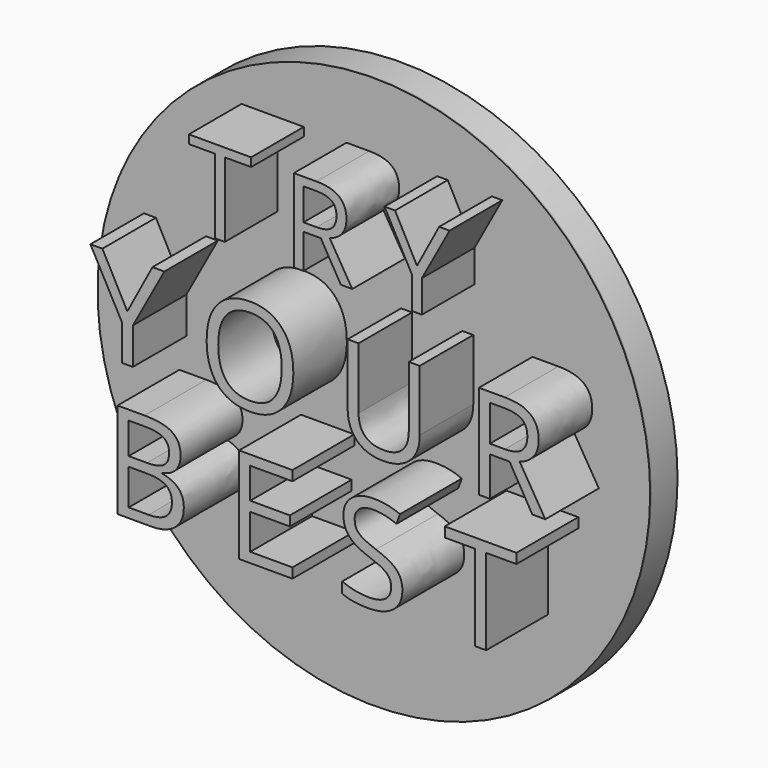
from build123d import *

# Parameters (mm, degrees)
F0_R         = 74.7496845117
F1_DEPTH     = 9.25076
F2_DEPTH     = 8.89276
F3_TEXT_SIZE = 31.4468880081
F6_DEPTH     = 17.81762
F4_TEXT_SIZE = 35.690900404
F7_DEPTH     = 18.10013
F5_TEXT_SIZE = 36.2257731871
F8_DEPTH     = 20.90356


# Not quite as in the source:
# - Text() gives the source's letters only with a copy of the font that has no kerning and outlines rounded to 1/6400 em; it was checked with that copy


with BuildPart() as f1:
    # F0 (on Front) → F1 (new body)
    with BuildSketch(Plane.XZ):
        Circle(F0_R)
    extrude(amount=-F1_DEPTH)

    # F2 (add): a face of the model
    f2_faces = [f1.faces().sort_by_distance(p)[0] for p in [
        (0, 9.25076, 0),
    ]]
    extrude(f2_faces, amount=-F2_DEPTH)

    # F3 (on face) → F6 (join)
    with BuildSketch(Plane.XZ):
        with Locations((-36.0579546541, 34.4763044268)):
            Text('T R Y', F3_TEXT_SIZE, font='Open Sans', text_align=(TextAlign.LEFT, TextAlign.BOTTOM))
    extrude(amount=F6_DEPTH)

    # F4 (on face) → F7 (join)
    with BuildSketch(Plane.XZ):
        with Locations((-62.1885545552, -3.1940236222)):
            Text('Y O U R', F4_TEXT_SIZE, font='Open Sans', text_align=(TextAlign.LEFT, TextAlign.BOTTOM))
    extrude(amount=F7_DEPTH)

    # F5 (on face) → F8 (join)
    with BuildSketch(Plane.XZ):
        with Locations((-56.1597375199, -37.7139672637)):
            Text('B E S T', F5_TEXT_SIZE, font='Open Sans', text_align=(TextAlign.LEFT, TextAlign.BOTTOM))
    extrude(amount=F8_DEPTH)


solid = f1.part
